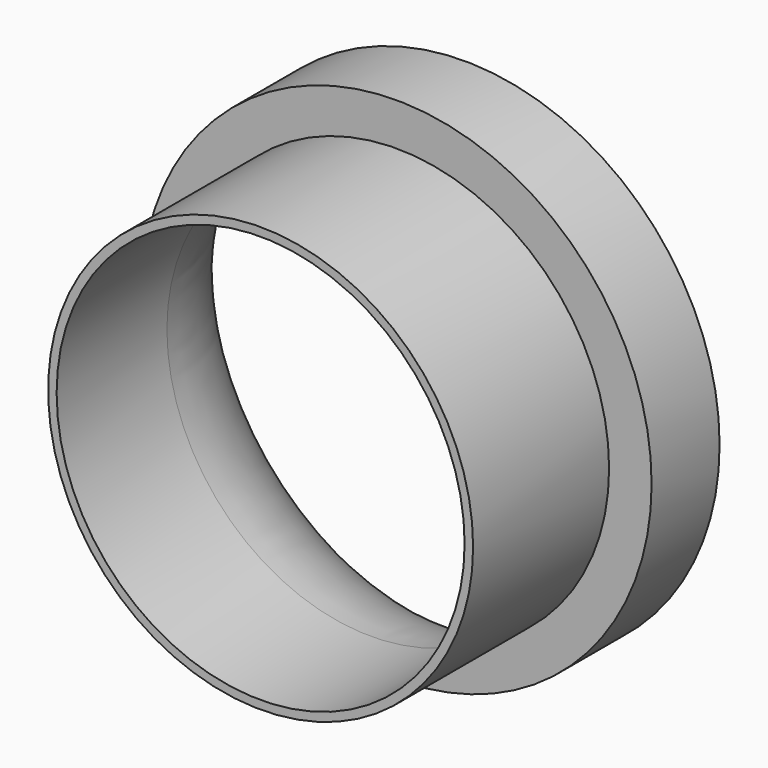
from build123d import *

# Parameters (mm, degrees)
F0_R     = 30
F1_DEPTH = 50
F2_R     = 30
F2_R_2   = 25
F3_DEPTH = 40
F4_R     = 24
F5_DEPTH = 60
F7_DEPTH = 20


# Not quite as in the source:
# - a fillet or chamfer that OpenCascade refuses, or shapes differently, is made with other operations: its cross-section is extruded or revolved along the edge and cut away or added


with BuildPart() as f1:
    # F0 (on Front) → F1 (new body)
    with BuildSketch(Plane.XZ):
        Circle(F0_R)
    extrude(amount=-F1_DEPTH)

    # F2 (on face) → F3 (cut)
    with BuildSketch(Plane.XZ):
        Circle(F2_R)
        Circle(F2_R_2, mode=Mode.SUBTRACT)
    extrude(amount=-F3_DEPTH, mode=Mode.SUBTRACT)

    # F4 (on face) → F5 (cut)
    with BuildSketch(Plane.XZ):
        Circle(F4_R)
    extrude(amount=-F5_DEPTH, mode=Mode.SUBTRACT)

    # F6: fillet of radius 18.8308657865 on 1 edges, made by hand

    # F6_s1 → F6_t2 (revolve, cut)
    with BuildSketch(Plane.XY):
        with BuildLine():
            ThreePointArc((30, 50), (25.5650351112, 43.7331811345), (24, 36.2170253777))
            Line((24, 36.2170253777), (23.6233826843, 36.2170253777))
            Line((23.6233826843, 36.2170253777), (23.6233826843, 50))
            Line((23.6233826843, 50), (24, 50.3766173157))
            ThreePointArc((24, 50.3766173157), (27, 50.3766173157), (29.7433826843, 50.2756594924))
            Line((29.7433826843, 50.2756594924), (30, 50))
        make_face()
    revolve(axis=Axis((0, 50, 0), (0, -1, 0)), mode=Mode.SUBTRACT)

    # F7 (cut): a face of the model
    f7_faces = [f1.faces().sort_by_distance(p)[0] for p in [
        (-24.2928932188, 0, 0),
    ]]
    extrude(f7_faces, amount=-F7_DEPTH, mode=Mode.SUBTRACT)


solid = f1.part
